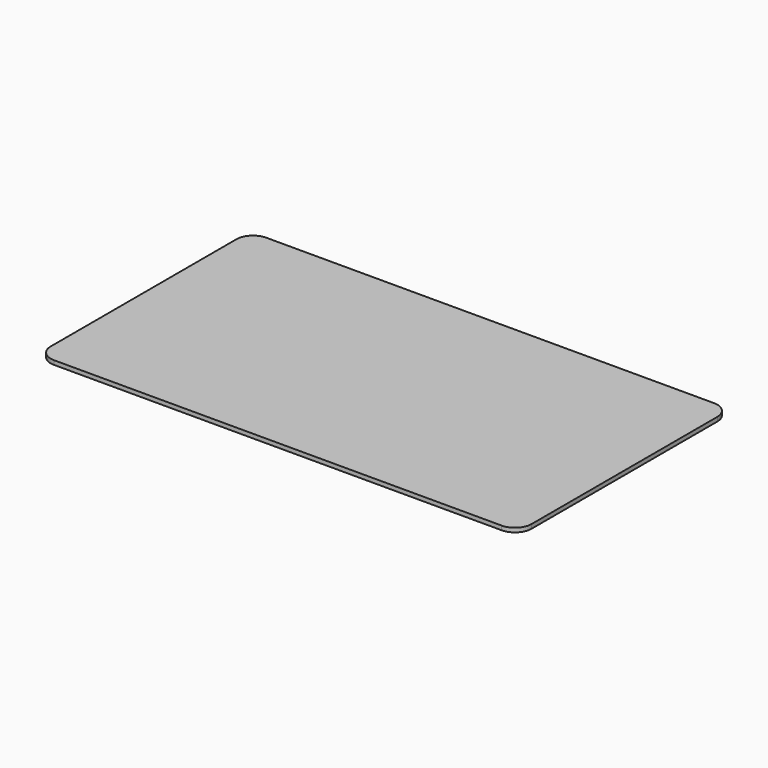
from build123d import *

# Parameters (mm, degrees)
F0_W     = 184.15
F0_H     = 101.6
F1_DEPTH = 1.5875
F2_R     = 6.35


# Not quite as in the source:
# - a length typed as a fraction of an inch, garbled in the dataset ("3 / 203.2 mm" for 3/8 in), is restored


with BuildPart() as f1:
    # F0 (on Top) → F1 (new body)
    with BuildSketch(Plane.XY):
        with Locations((92.075, 50.8)):
            Rectangle(F0_W, F0_H)
    extrude(amount=-F1_DEPTH)

    # F2
    f2_edges = [f1.edges().sort_by_distance(p)[0] for p in [
        (0, 101.6, -0.79375),
        (0, 0, -0.79375),
        (184.15, 0, -0.79375),
        (184.15, 101.6, -0.79375),
    ]]
    fillet(f2_edges, radius=F2_R)


solid = f1.part
